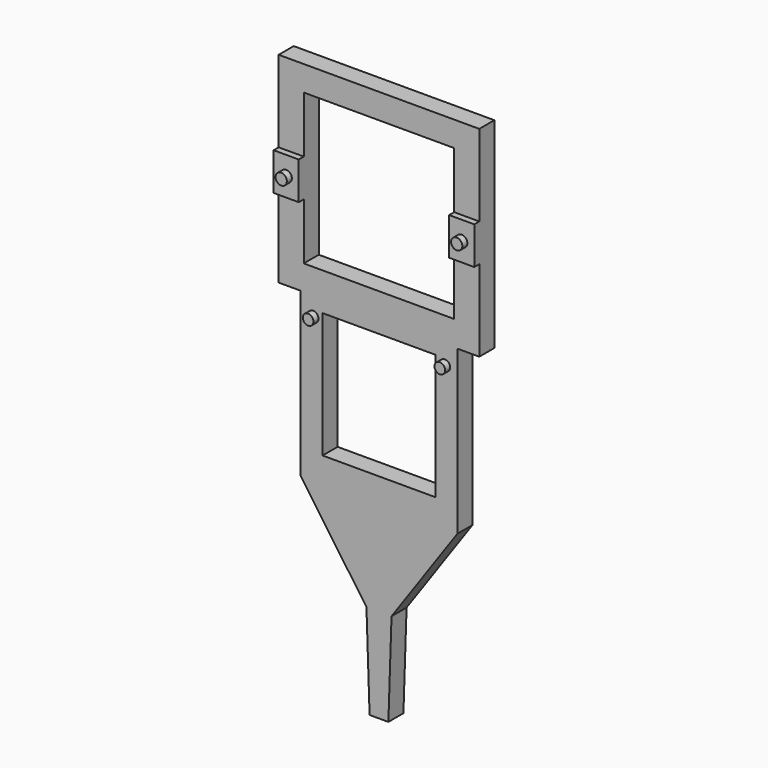
from build123d import *

# Parameters (mm, degrees)
F0_R     = 0.9
F1_DEPTH = 5
F0_R_2   = 0.85
F2_DEPTH = 4
F0_W     = 4
F0_H     = 6
F3_DEPTH = 4
F4_DEPTH = 3
F5_DEPTH = 3


# Not quite as in the source:
# - a feature names something its author has since deleted; it is built from what else it names


with BuildPart() as f1:
    # F0 (on Front) → F1 (new body)
    with BuildSketch(Plane.XZ):
        with Locations((-14, 12)):
            Circle(F0_R)
    extrude(amount=F1_DEPTH)

    # F0 (on Front) → F3 (join)
    with BuildSketch(Plane.XZ):
        with Locations((-14, 12)):
            Rectangle(F0_W, F0_H)
        with Locations((-14, 12)):
            Circle(F0_R, mode=Mode.SUBTRACT)
    extrude(amount=F3_DEPTH)



with BuildPart() as f1b:
    # F0 (on Front) → F1, piece 2 (new body)
    with BuildSketch(Plane.XZ):
        with Locations((14, 12)):
            Circle(F0_R)
    extrude(amount=F1_DEPTH)

    # F0 (on Front) → F3, piece 2 (join)
    with BuildSketch(Plane.XZ):
        with Locations((14, 12)):
            Rectangle(F0_W, F0_H)
        with Locations((14, 12)):
            Circle(F0_R, mode=Mode.SUBTRACT)
    extrude(amount=F3_DEPTH)


with BuildPart() as f2:
    # F0 (on Front) → F2 (new body)
    with BuildSketch(Plane.XZ):
        with Locations((-10.5, -7)):
            Circle(F0_R_2)
    extrude(amount=F2_DEPTH)


with BuildPart() as f2b:
    # F0 (on Front) → F2, piece 2 (new body)
    with BuildSketch(Plane.XZ):
        with Locations((10.5, -7)):
            Circle(F0_R_2)
    extrude(amount=F2_DEPTH)


with BuildPart() as f1_1:
    add(f1.part)

    add(f1b.part)  # F4 merges F1b

    add(f2.part)  # F4 merges F2

    add(f2b.part)  # F4 merges F2b
    # F0 (on Front) → F4 (join)
    with BuildSketch(Plane.XZ):
        Polygon((-12, 24), (0, 24), (0, 28), (-16, 28), (-16, 15), (-12, 15), align=None)
        Polygon((0, 28), (0, 24), (12, 24), (12, 15), (16, 15), (16, 28), align=None)
        Polygon((0, 0), (0, -4), (12.5, -4), (16, -4), (16, 9), (12, 9), (12, 0), align=None)
        Polygon((-16, -4), (-12.5, -4), (0, -4), (0, 0), (-12, 0), (-12, 9), (-16, 9), align=None)
        Polygon((0, -4), (-12.5, -4), (-12.5, -30), (0, -30), (0, -26), (-9, -26), (-9, -6), (0, -6), align=None)
        with Locations((-10.5, -7)):
            Circle(F0_R_2, mode=Mode.SUBTRACT)
        Polygon((12.5, -4), (0, -4), (0, -6), (9, -6), (9, -26), (0, -26), (0, -30), (12.5, -30), align=None)
        with Locations((10.5, -7)):
            Circle(F0_R_2, mode=Mode.SUBTRACT)
    extrude(amount=F4_DEPTH)

    # F0 (on Front) → F5 (join)
    with BuildSketch(Plane.XZ):
        Polygon((0, -30), (-12.5, -30), (-2, -45), (2, -45), (12.5, -30), align=None)
        Polygon((2, -45), (-2, -45), (-1.5, -60), (1.5, -60), align=None)
    extrude(amount=F5_DEPTH)


solid = f1_1.part
